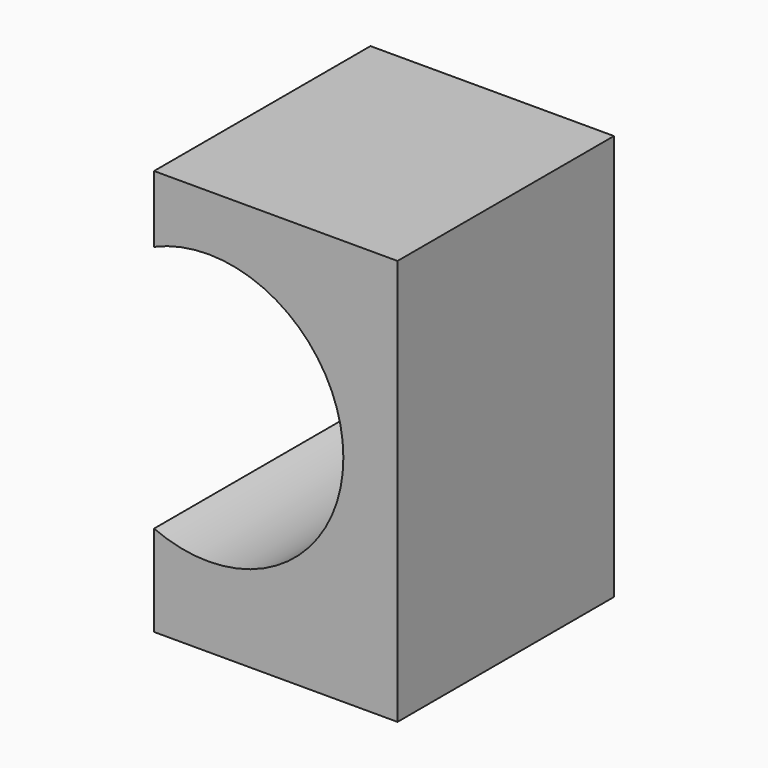
from build123d import *

# Parameters (mm, degrees)
F0_W     = 22.86
F0_H     = 38.1
F1_DEPTH = 25.4
F2_R     = 12.7
F3_DEPTH = 89
F5_DEPTH = 25.401


# Not quite as in the source:
# - an extrude ends at something that could not be found from the text; its depth is read off the source's solid


with BuildPart() as f1:
    # F0 (on Front) → F1 (new body)
    with BuildSketch(Plane.XZ):
        with Locations((-34.8423583888, -1.1378988595)):
            Rectangle(F0_W, F0_H)
    extrude(amount=F1_DEPTH)

    # F2 (on Front) → F3 (cut, through all)
    with BuildSketch(Plane.XZ):
        with Locations((-35.3627614677, 3.7935657892)):
            Circle(F2_R)
    extrude(amount=-F3_DEPTH, mode=Mode.SUBTRACT)

    # F4 (on face) → F5 (cut, through all)
    with BuildSketch(Plane(origin=(0, 0, 0), x_dir=(-1, 0, 0), z_dir=(0, 1, 0))):
        with BuildLine():
            ThreePointArc((46.2723583888, -11.6417417865), (51.8211548639, -6.9581684388), (53.8969423294, 0))
            ThreePointArc((53.8969423294, 0), (51.8211548639, 6.9581684388), (46.2723583888, 11.6417417865))
            Line((46.2723583888, 11.6417417865), (46.2723583888, -11.6417417865))
        make_face()
        with BuildLine():
            Line((46.2723583888, -11.6417417865), (46.2723583888, 11.6417417865))
            ThreePointArc((46.2723583888, 11.6417417865), (28.4969423294, 0), (46.2723583888, -11.6417417865))
        make_face()
    extrude(amount=-F5_DEPTH, mode=Mode.SUBTRACT)


solid = f1.part
